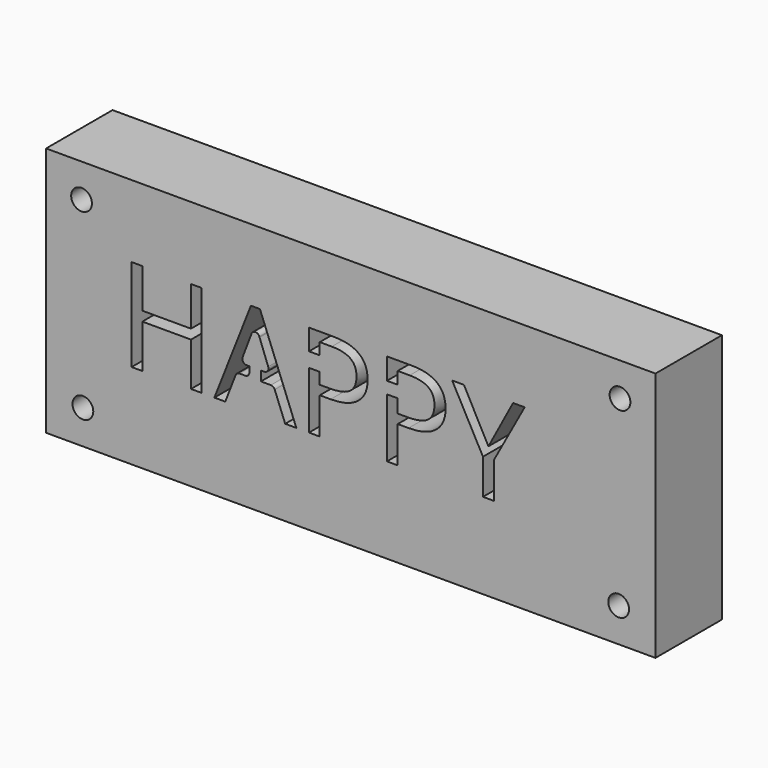
from build123d import *

# Parameters (mm, degrees)
F0_W         = 186.3412410021
F0_H         = 76.5538960695
F1_DEPTH     = 25.4
F2_TEXT_SIZE = 39.587489381
F3_DEPTH     = 0.0254
F4_W         = 3.520526767
F4_H         = 6.1620473688
F4_W_2       = 10.5363738484
F4_H_2       = 4.4442722574
F4_W_3       = 10.1218921728
F4_H_3       = 3.6407969892
F5_DEPTH     = 5.08
F6_DEPTH     = 25.4
F7_T1_DEPTH  = 29.7328547206
F7_T3_DEPTH  = 34.5691133359
F7_T5_DEPTH  = 35.5308624579
F7_T7_DEPTH  = 10.1816624579
F7_T9_DEPTH  = 34.599454084
F7_T11_DEPTH = 25.4
F7_T13_DEPTH = 29.7523511372
F8_R         = 3.175
F9_DEPTH     = 25.4


# Not quite as in the source:
# - a fillet or chamfer that OpenCascade refuses, or shapes differently, is made with other operations: its cross-section is extruded or revolved along the edge and cut away or added
# - Text() gives the source's letters only with a copy of the font that has no kerning and outlines rounded to 1/6400 em; it was checked with that copy


with BuildPart() as f1:
    # F0 (on Front) → F1 (new body)
    with BuildSketch(Plane.XZ):
        Rectangle(F0_W, F0_H)
    extrude(amount=F1_DEPTH)

    # F2 (on face) → F3 (cut)
    with BuildSketch(Plane.XZ.offset(25.4)):
        with Locations((-70.9153339267, -12.0686208829)):
            Text('HAPPY', F2_TEXT_SIZE, font='Open Sans', text_align=(TextAlign.LEFT, TextAlign.BOTTOM))
    extrude(amount=-F3_DEPTH, mode=Mode.SUBTRACT)

    # F4 (on face) → F5 (join)
    with BuildSketch(Plane.XZ.offset(25.4)):
        with Locations((-29.2402230353, -3.0810236844)):
            Rectangle(F4_W, F4_H)
        with Locations((-12.7712088983, 7.577625569)):
            Rectangle(F4_W_2, F4_H_2)
        with Locations((11.0616968181, 7.8052966855)):
            Rectangle(F4_W_3, F4_H_3)
    extrude(amount=-F5_DEPTH)

    # F6 (cut): faces of the model
    f6_faces = [f1.faces().sort_by_distance(p)[0] for p in [
        (-56.3019833544, -25.3746, 2.1837503825),
        (-25.5286580211, -25.3746, -2.70247921),
        (4.8032585578, -25.3746, 7.4622397253),
        (28.6361642742, -25.3746, 7.4622397253),
        (46.1723614395, -25.3746, 8.9571901275),
    ]]
    extrude(f6_faces, amount=-F6_DEPTH, mode=Mode.SUBTRACT)

    # F7: fillet of radius 1.27 on 7 edges, made by hand

    # F7_s2 → F7_t1 (cut)
    with BuildSketch(Plane.XZ.offset(-2.1664273603)):
        with BuildLine():
            ThreePointArc((-24.4439273344, -3.0810236844), (-23.7281164009, -3.3019694878), (-23.2613691237, -3.8879296569))
            Line((-23.2613691237, -3.8879296569), (-23.2377179595, -3.8786677764))
            Line((-23.2377179595, -3.8786677764), (-23.5600249714, -3.0556236844))
            Line((-23.5600249714, -3.0556236844), (-24.4439273344, -3.0556236844))
            Line((-24.4439273344, -3.0556236844), (-24.4439273344, -3.0810236844))
        make_face()
    extrude(amount=F7_T1_DEPTH, mode=Mode.SUBTRACT)

    # F7_s4 → F7_t3 (cut)
    with BuildSketch(Plane.XZ.offset(-4.5845566679)):
        with BuildLine():
            ThreePointArc((-25.2429322205, 1.5923296945), (-25.3877246448, 0.4226045914), (-26.4317940181, -0.1243330712))
            Line((-26.4317940181, -0.1243330712), (-26.4317940181, -0.1497330712))
            Line((-26.4317940181, -0.1497330712), (-24.5612948975, -0.1497330712))
            Line((-24.5612948975, -0.1497330712), (-25.2191549846, 1.6012629498))
            Line((-25.2191549846, 1.6012629498), (-25.2429322205, 1.5923296945))
        make_face()
    extrude(amount=F7_T3_DEPTH, mode=Mode.SUBTRACT)

    # F7_s6 → F7_t5 (cut)
    with BuildSketch(Plane.XZ.offset(-10.1562624579)):
        with BuildLine():
            ThreePointArc((-30.3538887272, 8.8169280821), (-29.1682549755, 9.6650246118), (-27.9664698085, 8.8399745955))
            Line((-27.9664698085, 8.8399745955), (-27.942679288, 8.8488724118))
            ThreePointArc((-27.942679288, 8.8488724118), (-28.599121103, 10.7703201096), (-29.1755544509, 12.717510218))
            Line((-29.1755544509, 12.717510218), (-29.2247706932, 12.7163666029))
            ThreePointArc((-29.2247706932, 12.7163666029), (-29.7472238687, 10.7548987689), (-30.3778465851, 8.8253649681))
            Line((-30.3778465851, 8.8253649681), (-30.3538887272, 8.8169280821))
        make_face()
    extrude(amount=F7_T5_DEPTH, mode=Mode.SUBTRACT)

    # F7_s8 → F7_t7 (cut)
    with BuildSketch(Plane.XZ.offset(25.3746)):
        with BuildLine():
            ThreePointArc((-30.3538887272, 8.8169280821), (-29.1682549755, 9.6650246118), (-27.9664698085, 8.8399745955))
            Line((-27.9664698085, 8.8399745955), (-27.942679288, 8.8488724118))
            ThreePointArc((-27.942679288, 8.8488724118), (-28.599121103, 10.7703201096), (-29.1755544509, 12.717510218))
            Line((-29.1755544509, 12.717510218), (-29.2247706932, 12.7163666029))
            ThreePointArc((-29.2247706932, 12.7163666029), (-29.7472238687, 10.7548987689), (-30.3778465851, 8.8253649681))
            Line((-30.3778465851, 8.8253649681), (-30.3538887272, 8.8169280821))
        make_face()
    extrude(amount=F7_T7_DEPTH, mode=Mode.SUBTRACT)

    # F7_s10 → F7_t9 (cut)
    with BuildSketch(Plane.XZ.offset(-4.599727042)):
        with BuildLine():
            ThreePointArc((-31.900316363, -0.1243330712), (-32.9455018716, 0.4242189038), (-33.0877919864, 1.5960019639))
            Line((-33.0877919864, 1.5960019639), (-33.1115414989, 1.6050086646))
            Line((-33.1115414989, 1.6050086646), (-33.7770049962, -0.1497330712))
            Line((-33.7770049962, -0.1497330712), (-31.900316363, -0.1497330712))
            Line((-31.900316363, -0.1497330712), (-31.900316363, -0.1243330712))
        make_face()
    extrude(amount=F7_T9_DEPTH, mode=Mode.SUBTRACT)

    # F7_s12 → F7_t11 (join)
    with BuildSketch(Plane.XZ):
        with BuildLine():
            ThreePointArc((-32.2704864188, -3.0810236844), (-31.3724608067, -2.7090492965), (-31.0004864188, -1.8110236844))
            Line((-31.0004864188, -1.8110236844), (-30.9750864188, -1.8110236844))
            Line((-30.9750864188, -1.8110236844), (-30.9750864188, -3.1064236844))
            Line((-30.9750864188, -3.1064236844), (-32.2704864188, -3.1064236844))
            Line((-32.2704864188, -3.1064236844), (-32.2704864188, -3.0810236844))
        make_face()
    extrude(amount=F7_T11_DEPTH)

    # F7_s14 → F7_t13 (cut)
    with BuildSketch(Plane.XZ.offset(-2.1761755686)):
        with BuildLine():
            ThreePointArc((-35.2171048343, -3.8928813689), (-34.7506233733, -3.3034692131), (-34.0326194529, -3.0810236844))
            Line((-34.0326194529, -3.0810236844), (-34.0326194529, -3.0556236844))
            Line((-34.0326194529, -3.0556236844), (-34.9204990849, -3.0556236844))
            Line((-34.9204990849, -3.0556236844), (-35.240794542, -3.8837185226))
            Line((-35.240794542, -3.8837185226), (-35.2171048343, -3.8928813689))
        make_face()
    extrude(amount=F7_T13_DEPTH, mode=Mode.SUBTRACT)

    # F8 (on face) → F9 (cut)
    with BuildSketch(Plane.XZ.offset(25.4)):
        with Locations((-81.915, -27.8587673865)):
            Circle(F8_R)
        with Locations((-82.3219577746, 28.0197507163)):
            Circle(F8_R)
        with Locations((81.915, -27.8587673865)):
            Circle(F8_R)
        with Locations((82.3219577746, 28.0197507163)):
            Circle(F8_R)
    extrude(amount=-F9_DEPTH, mode=Mode.SUBTRACT)


solid = f1.part
